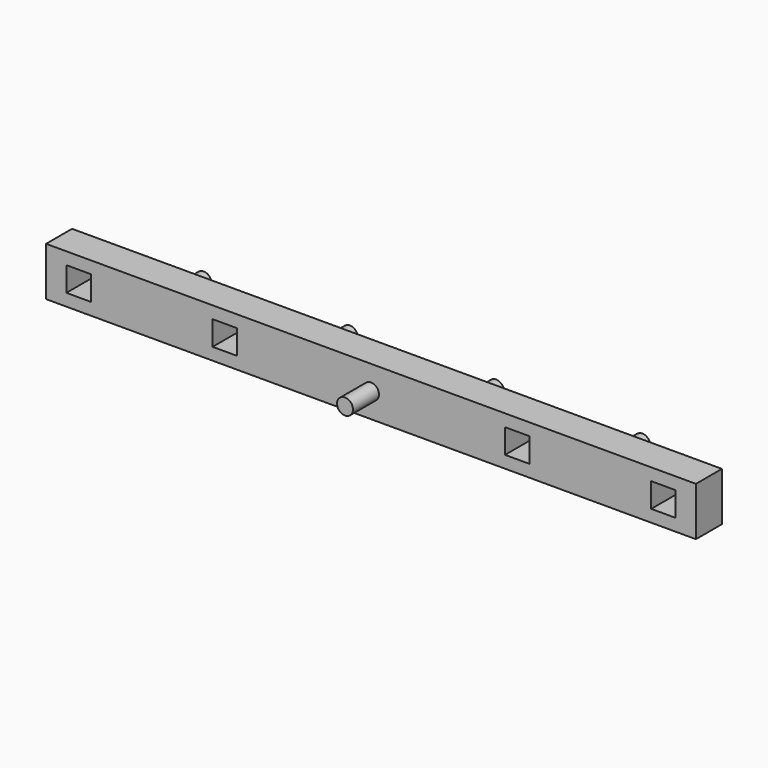
from build123d import *

# Parameters (mm, degrees)
F0_W     = 254
F0_H     = 19.05
F1_DEPTH = 12.7
F2_R     = 3.1115
F3_DEPTH = 12.7
F4_W     = 9.525
F4_H     = 9.525
F4_R     = 3.1115
F5_DEPTH = 12.7
F6_DEPTH = 25.4


# Not quite as in the source:
# - a feature names something its author has since deleted; it is built from what else it names


with BuildPart() as f1:
    # F0 (on Front) → F1 (new body)
    with BuildSketch(Plane.XZ):
        Rectangle(F0_W, F0_H)
    extrude(amount=F1_DEPTH)

    # F2 (on face) → F3 (join)
    with BuildSketch(Plane.XZ.offset(12.7)):
        Circle(F2_R)
    extrude(amount=F3_DEPTH)

    # F4 (on face) → F5 (join)
    with BuildSketch(Plane(origin=(0, 0, 0), x_dir=(-1, 0, 0), z_dir=(0, 1, 0))):
        with Locations((-114.3, 0)):
            Rectangle(F4_W, F4_H)
        with Locations((-85.725, 0)):
            Circle(F4_R)
        with Locations((-57.15, 0)):
            Rectangle(F4_W, F4_H)
        with Locations((-28.575, 0)):
            Circle(F4_R)
        with Locations((28.575, 0)):
            Circle(F4_R)
        with Locations((57.15, 0)):
            Rectangle(F4_W, F4_H)
        with Locations((85.725, 0)):
            Circle(F4_R)
        with Locations((114.3, 0)):
            Rectangle(F4_W, F4_H)
    extrude(amount=F5_DEPTH)

    # F6 (cut): faces of the model
    f6_faces = [f1.faces().sort_by_distance(p)[0] for p in [
        (114.3, 12.7, 0),
        (57.15, 12.7, 0),
        (-57.15, 12.7, 0),
        (-114.3, 12.7, 0),
    ]]
    extrude(f6_faces, amount=-F6_DEPTH, mode=Mode.SUBTRACT)


solid = f1.part
